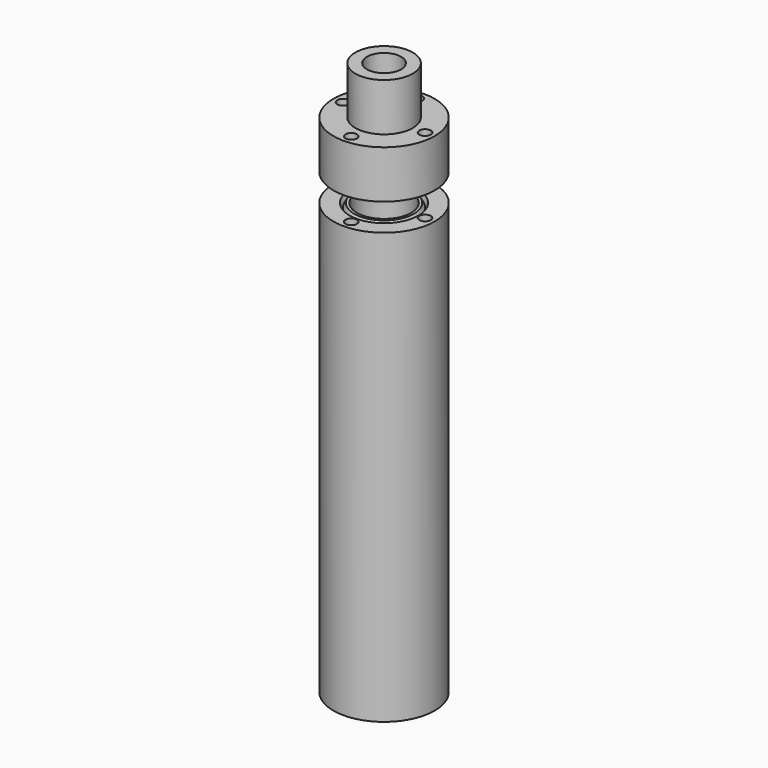
from build123d import *

# Parameters (mm, degrees)
F1_W     = 5.08
F1_H     = 80
F4_D     = 2.1336
F4_DEPTH = 25.4
F4_TIP   = 0.6409981084
F5_D     = 2.1336
F6_D     = 10.0838
F6_DEPTH = 72.39
F6_TIP   = 3.0294791551


# Not quite as in the source:
# - a feature names something its author has since deleted; it is built from what else it names


with BuildPart() as f2:
    # F1 (on Front) → F2 (revolve)
    with BuildSketch(Plane.XZ):
        Polygon((9.398, -90.0780827382), (9.398, -10.0780827382), (6.3953505707, -10.0780827382), (5.969, -10.8400827382), (5.5426494293, -10.0780827382), (5.08, -10.0780827382), (5.08, -90.0780827382), align=None)
        with Locations((2.54, -50.0780827382)):
            Rectangle(F1_W, F1_H)
    revolve(axis=Axis((0, 0, -0.125199824), (0, 0, -1)))

    # F4
    with Locations(Plane.XY.offset(-10.0780827382)):
        with Locations((-7.62, 0), (0, 7.62), (7.62, 0), (0, -7.62)):
            Hole(F4_D / 2, depth=F4_DEPTH)
            with Locations((0, 0, -(F4_DEPTH + F4_TIP / 2))):  # 118° drill point
                Cone(0, F4_D / 2, F4_TIP, mode=Mode.SUBTRACT)

    # F6
    with Locations(Plane.XY.offset(-10.0780827382)):
        with Locations((0, 0)):
            Hole(F6_D / 2, depth=F6_DEPTH)
            with Locations((0, 0, -(F6_DEPTH + F6_TIP / 2))):  # 118° drill point
                Cone(0, F6_D / 2, F6_TIP, mode=Mode.SUBTRACT)


with BuildPart() as f2b:
    # F1 (on Front) → F2, piece 2 (revolve)
    with BuildSketch(Plane.XZ):
        Polygon((5.334, 3.8919172618), (5.334, 12.7819172618), (3.175, 12.7819172618), (3.175, 6.4319172618), (1.143, 6.4319172618), (1.143, -4.9980827382), (9.398, -4.9980827382), (9.398, 3.8919172618), align=None)
    revolve(axis=Axis((0, 0, -0.125199824), (0, 0, -1)))

    # F5 (through all)
    with Locations(Plane(origin=(0, 0, -10.0780827382), x_dir=(1, 0, 0), z_dir=(0, 0, -1))):
        with Locations((0, 7.62), (7.62, 0), (0, -7.62), (-7.62, 0)):
            Hole(F5_D / 2)


solid = Compound([f2.part, f2b.part])
